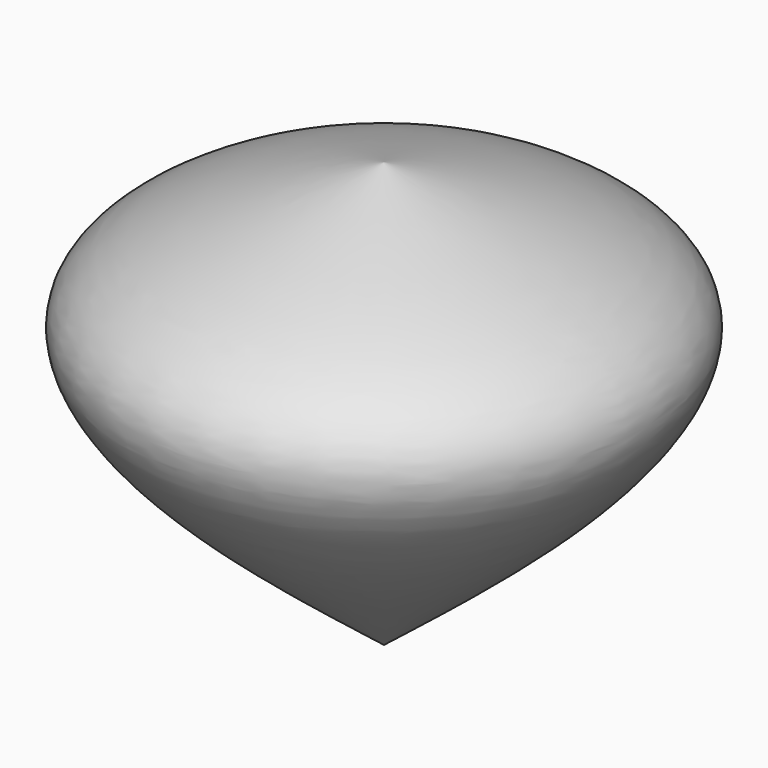
from build123d import *


# Not quite as in the source:
# - the program builds the solid bodies; features that only make, move or delete a surface that nothing else refers to are left out


with BuildPart() as f1:
    # F0 (on Front) → F1 (revolve)
    with BuildSketch(Plane.XZ):
        with BuildLine():
            Line((0, 20.6253648025), (0, 0))
            add(Edge.make_bspline(
                [(0, 0), (13.5426130018, 10.6561129629), (31.7562955237, 24.9876942019), (23.1282978753, 32.9251076368), (19.8509394438, 34.7071183581)],
                knots=[0, 0, 0, 0, 0.5350714955, 0.7196264373, 0.7196264373, 0.7196264373, 0.7196264373], degree=3))
            ThreePointArc((19.8509394438, 34.7071183581), (12.1691780741, 24.5033032109), (0, 20.6253648025))
        make_face()
        with BuildLine():
            Line((0, 41.6580997407), (0, 20.6253648025))
            ThreePointArc((0, 20.6253648025), (12.1691780741, 24.5033032109), (19.8509394438, 34.7071183581))
            add(Edge.make_bspline(
                [(19.8509394438, 34.7071183581), (14.8720174437, 37.4143267914), (7.4360087219, 39.5362132661), (0, 41.6580997407)],
                knots=[0.7196264373, 0.7196264373, 0.7196264373, 0.7196264373, 1, 1, 1, 1], degree=3))
        make_face()
    revolve(axis=Axis((0, 0, 20.8290498704), (0, 0, 1)))


solid = f1.part
